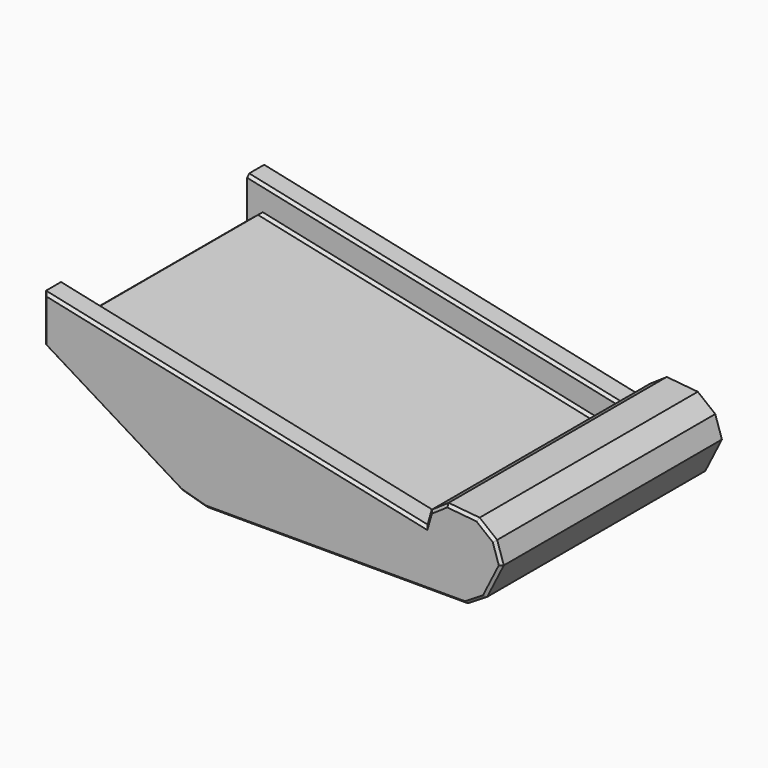
from build123d import *

# Parameters (mm, degrees)
F1_DEPTH      = 52
F1_DEPTH_BACK = 52
F2_W          = 173.7792565062
F2_H          = 86
F2_W_2        = 146
F3_DEPTH      = 10
F4_TEXT_SIZE  = 49.8597693986
F5_DEPTH      = 3
F6_SIZE       = 5
F7_SIZE       = 5
F8_SIZE       = 5
F9_SIZE       = 5
F10_SIZE      = 5
F11_SIZE      = 1
F12_SIZE      = 1
F13_SIZE      = 1


# Not quite as in the source:
# - Text() gives the source's letters only with a copy of the font that has no kerning and outlines rounded to 1/6400 em; it was checked with that copy


with BuildPart() as f1:
    # F0 (on Front) → F1 (new body, two sides)
    with BuildSketch(Plane.XZ) as f1_sk:
        Polygon((52.6875165238, -12.9319923499), (-90.0624310977, 17.7021789965), (-90.0624310977, 0), (-34.6387099491, -33.9589624996), (72.7452889392, -33.9589624996), (81.1989820422, -17.0948275187), (77.1373834181, -4.7848284553), (55.5867925608, -2.7331863087), align=None)
    extrude(amount=F1_DEPTH)
    extrude(f1_sk.sketch, amount=-F1_DEPTH_BACK)

    # F2 (on face) → F3 (cut)
    with BuildSketch(Plane(origin=(-0.3334215701, 0, -1.5536869313), x_dir=(0.9777393673, 0, -0.2098230914), z_dir=(0.2098230914, 0, 0.9777393673))):
        with Locations((-32.6615385711, 0)):
            Rectangle(F2_W, F2_H)
        with Locations((-18.771910318, 0)):
            Rectangle(F2_W_2, F2_H)
    extrude(amount=-F3_DEPTH, mode=Mode.SUBTRACT)

    # F4 (on face) → F5 (cut)
    with BuildSketch(Plane(origin=(-24.582484805, 0, -40.1205656088), x_dir=(0.8526726331, 0, -0.5224455769), z_dir=(-0.5224455769, 0, -0.8526726331))):
        with Locations((-65.388784145, -18.5934174644)):
            Text('JB', F4_TEXT_SIZE, font='Open Sans', text_align=(TextAlign.LEFT, TextAlign.BOTTOM))
    extrude(amount=-F5_DEPTH, mode=Mode.SUBTRACT)

    # F6
    f6_edges = [f1.edges().sort_by_distance(p)[0] for p in [
        (77.137383, 0, -4.784828),
    ]]
    chamfer(f6_edges, length=F6_SIZE)

    # F7
    f7_edges = [f1.edges().sort_by_distance(p)[0] for p in [
        (55.586793, 0, -2.733186),
    ]]
    chamfer(f7_edges, length=F7_SIZE)

    # F8
    f8_edges = [f1.edges().sort_by_distance(p)[0] for p in [
        (72.745289, 0, -33.958962),
    ]]
    chamfer(f8_edges, length=F8_SIZE)

    # F9
    f9_edges = [f1.edges().sort_by_distance(p)[0] for p in [
        (-90.062431, 0, 7.474504),
    ]]
    chamfer(f9_edges, length=F9_SIZE)

    # F10
    f10_edges = [f1.edges().sort_by_distance(p)[0] for p in [
        (-34.63871, 0, -33.958962),
    ]]
    chamfer(f10_edges, length=F10_SIZE)

    # F11
    f11_edges = [f1.edges().sort_by_distance(p)[0] for p in [
        (19.053289, -52, -33.958962),
        (-34.270392, -52, -32.652849),
        (71.365615, -52, -31.724042),
        (-64.482252, -52, -15.673367),
        (78.092462, -52, -23.291975),
        (-90.062431, -52, 8.851089),
        (79.951504, -52, -13.31394),
        (-18.687457, -52, 2.385093),
        (75.431958, -52, -6.922009),
        (53.45355, -52, -10.237311),
        (66.362088, -52, -3.759007),
        (57.391935, -52, -5.374839),
    ]]
    chamfer(f11_edges, length=F11_SIZE)

    # F12
    f12_edges = [f1.edges().sort_by_distance(p)[0] for p in [
        (19.053289, 52, -33.958962),
        (-34.270392, 52, -32.652849),
        (71.365615, 52, -31.724042),
        (-64.482252, 52, -15.673367),
        (78.092462, 52, -23.291975),
        (-90.062431, 52, 8.851089),
        (79.951504, 52, -13.31394),
        (-18.687457, 52, 2.385093),
        (75.431958, 52, -6.922009),
        (53.45355, 52, -10.237311),
        (66.362088, 52, -3.759007),
        (57.391935, 52, -5.374839),
    ]]
    chamfer(f12_edges, length=F12_SIZE)

    # F13
    f13_edges = [f1.edges().sort_by_distance(p)[0] for p in [
        (-17.292224, 43, -8.141998),
        (-18.687457, 43, 2.385093),
        (-17.292224, -43, -8.141998),
        (-18.687457, -43, 2.385093),
    ]]
    chamfer(f13_edges, length=F13_SIZE)


solid = f1.part
